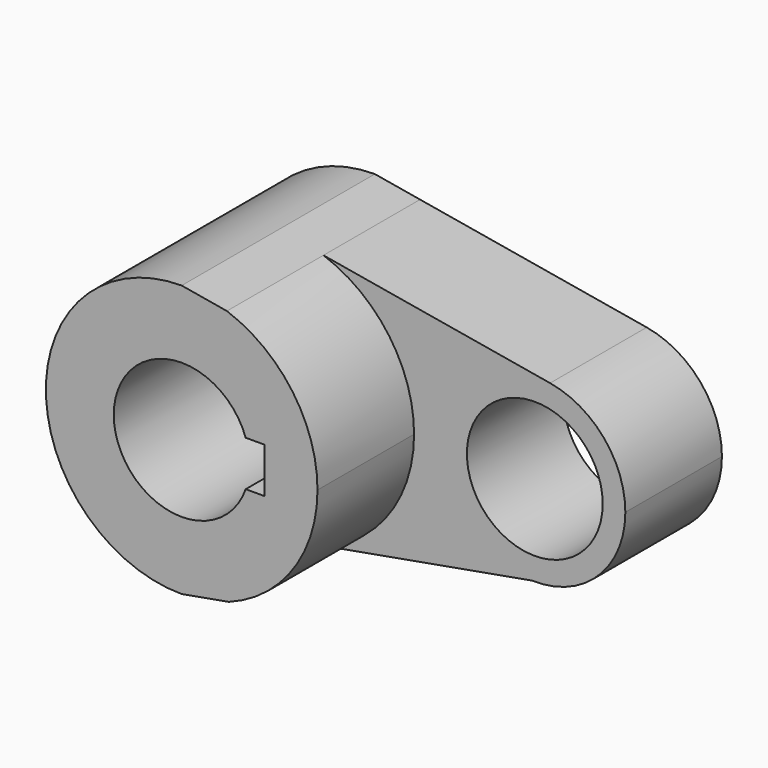
from build123d import *

# Parameters (mm, degrees)
F0_R     = 14.2875
F1_DEPTH = 25.4
F2_DEPTH = 50.8


with BuildPart() as f1:
    # F0 (on Front) → F1 (new body)
    with BuildSketch(Plane.XZ):
        with BuildLine():
            Line((9.5121844836, 26.9452959039), (0, 28.575))
            ThreePointArc((0, 28.575), (-28.575, 0), (0, -28.575))
            Line((0, -28.575), (9.8913467837, -26.8084293424))
            ThreePointArc((9.8913467837, -26.8084293424), (23.4432917841, -16.3383810498), (28.575, 0))
            ThreePointArc((28.575, 0), (23.3274655355, 16.5033322905), (9.5121844836, 26.9452959039))
        make_face()
        with BuildLine():
            ThreePointArc((-13.4703841816, 4.7625), (0, 14.2875), (13.4703841816, 4.7625))
            Line((13.4703841816, 4.7625), (17.3846837133, 4.7625))
            Line((17.3846837133, 4.7625), (17.3846837133, -4.7625))
            Line((17.3846837133, -4.7625), (13.4703841816, -4.7625))
            ThreePointArc((13.4703841816, -4.7625), (0, -14.2875), (-13.4703841816, -4.7625))
            Line((-13.4703841816, -4.7625), (-17.3846837133, -4.7625))
            Line((-17.3846837133, -4.7625), (-17.3846837133, 4.7625))
            Line((-17.3846837133, 4.7625), (-13.4703841816, 4.7625))
        make_face(mode=Mode.SUBTRACT)
        with BuildLine():
            Line((57.1919272622, 18.7764181619), (9.5121844836, 26.9452959039))
            ThreePointArc((9.5121844836, 26.9452959039), (23.3274655355, 16.5033322905), (28.575, 0))
            ThreePointArc((28.575, 0), (23.4432917841, -16.3383810498), (9.8913467837, -26.8084293424))
            Line((9.8913467837, -26.8084293424), (53.3836000765, -19.0408178955))
            ThreePointArc((53.3836000765, -19.0408178955), (35.0208663029, 1.9087471789), (57.1919272622, 18.7764181619))
        make_face()
        with BuildLine():
            ThreePointArc((73.025, 0), (68.5383952831, 12.2804730295), (57.1919272622, 18.7764181619))
            ThreePointArc((57.1919272622, 18.7764181619), (35.0208663029, 1.9087471789), (53.3836000765, -19.0408178955))
            ThreePointArc((53.3836000765, -19.0408178955), (67.2346442535, -13.67787755), (73.025, 0))
        make_face()
        with Locations((53.975, 0)):
            Circle(F0_R, mode=Mode.SUBTRACT)
        with BuildLine():
            ThreePointArc((-13.4703841816, -4.7625), (-14.2875, 0), (-13.4703841816, 4.7625))
            Line((-13.4703841816, 4.7625), (-17.3846837133, 4.7625))
            Line((-17.3846837133, 4.7625), (-17.3846837133, -4.7625))
            Line((-17.3846837133, -4.7625), (-13.4703841816, -4.7625))
        make_face()
    extrude(amount=F1_DEPTH)

    # F0 (on Front) → F2 (join)
    with BuildSketch(Plane.XZ):
        with BuildLine():
            Line((9.5121844836, 26.9452959039), (0, 28.575))
            ThreePointArc((0, 28.575), (-28.575, 0), (0, -28.575))
            Line((0, -28.575), (9.8913467837, -26.8084293424))
            ThreePointArc((9.8913467837, -26.8084293424), (23.4432917841, -16.3383810498), (28.575, 0))
            ThreePointArc((28.575, 0), (23.3274655355, 16.5033322905), (9.5121844836, 26.9452959039))
        make_face()
        with BuildLine():
            ThreePointArc((-13.4703841816, 4.7625), (0, 14.2875), (13.4703841816, 4.7625))
            Line((13.4703841816, 4.7625), (17.3846837133, 4.7625))
            Line((17.3846837133, 4.7625), (17.3846837133, -4.7625))
            Line((17.3846837133, -4.7625), (13.4703841816, -4.7625))
            ThreePointArc((13.4703841816, -4.7625), (0, -14.2875), (-13.4703841816, -4.7625))
            Line((-13.4703841816, -4.7625), (-17.3846837133, -4.7625))
            Line((-17.3846837133, -4.7625), (-17.3846837133, 4.7625))
            Line((-17.3846837133, 4.7625), (-13.4703841816, 4.7625))
        make_face(mode=Mode.SUBTRACT)
        with BuildLine():
            ThreePointArc((-13.4703841816, -4.7625), (-14.2875, 0), (-13.4703841816, 4.7625))
            Line((-13.4703841816, 4.7625), (-17.3846837133, 4.7625))
            Line((-17.3846837133, 4.7625), (-17.3846837133, -4.7625))
            Line((-17.3846837133, -4.7625), (-13.4703841816, -4.7625))
        make_face()
    extrude(amount=F2_DEPTH)


solid = f1.part
